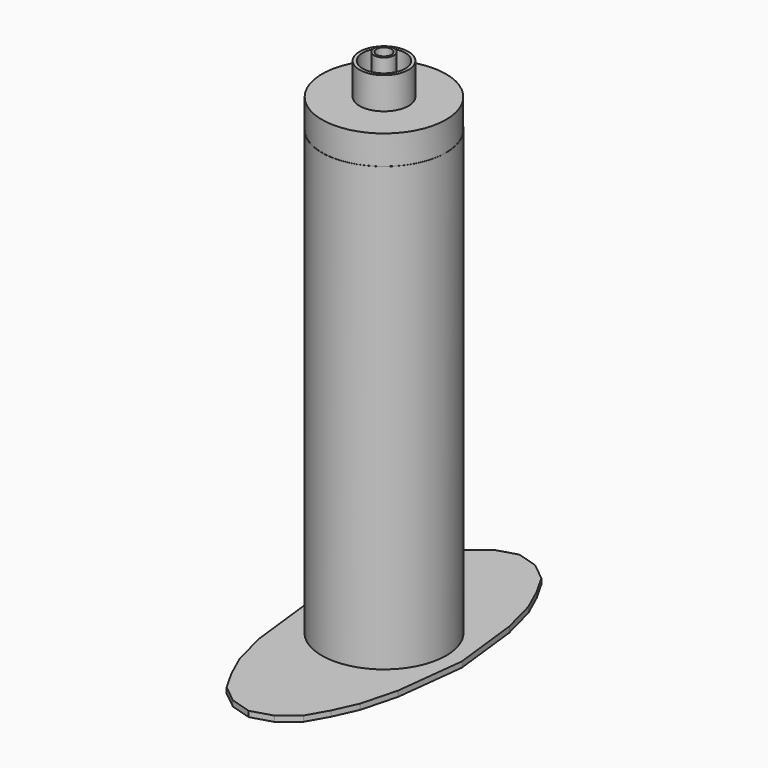
from build123d import *

# Parameters (mm, degrees)
F0_R      = 28.3177523181
F1_DEPTH  = 141.224
F2_DEPTH  = 60.452
F3_R      = 26.2473166526
F4_DEPTH  = 198.628
F5_R      = 28.3177523181
F6_DEPTH  = 2.54
F7_R      = 28.2282534547
F8_DEPTH  = 13.208
F9_R      = 11.1815753047
F10_DEPTH = 14.478
F11_R     = 9.7009276287
F12_DEPTH = 13.462
F13_R     = 4.462331727
F14_DEPTH = 14.478
F15_DEPTH = 3.556
F16_R     = 3.4559757879
F17_DEPTH = 18.034


# Not quite as in the source:
# - a feature names something its author has since deleted; it is built from what else it names


with BuildPart() as f1:
    # F0 (on Top) → F1 (new body)
    with BuildSketch(Plane.XY):
        Circle(F0_R)
    extrude(amount=F1_DEPTH)

    # F2 (add): a face of the model
    f2_faces = [f1.faces().sort_by_distance(p)[0] for p in [
        (0, 0, 0),
    ]]
    extrude(f2_faces, amount=F2_DEPTH)

    # F3 (on face) → F4 (cut)
    with BuildSketch(Plane(origin=(0, 0, -60.452), x_dir=(1, 0, 0), z_dir=(0, 0, -1))):
        Circle(F3_R)
    extrude(amount=-F4_DEPTH, mode=Mode.SUBTRACT)

    # F7 (on face) → F8 (join)
    with BuildSketch(Plane.XY.offset(141.224)):
        Circle(F7_R)
    extrude(amount=F8_DEPTH)

    # F9 (on face) → F10 (join)
    with BuildSketch(Plane.XY.offset(154.432)):
        Circle(F9_R)
    extrude(amount=F10_DEPTH)

    # F11 (on face) → F12 (cut)
    with BuildSketch(Plane.XY.offset(168.91)):
        Circle(F11_R)
    extrude(amount=-F12_DEPTH, mode=Mode.SUBTRACT)

    # F13 (on face) → F14 (join)
    with BuildSketch(Plane.XY.offset(168.91)):
        Circle(F13_R)
    extrude(amount=-F14_DEPTH)

    # F15 (add): a face of the model
    f15_faces = [f1.faces().sort_by_distance(p)[0] for p in [
        (0, 0, 168.91),
    ]]
    extrude(f15_faces, amount=F15_DEPTH)

    # F16 (on face) → F17 (cut)
    with BuildSketch(Plane.XY.offset(172.466)):
        Circle(F16_R)
    extrude(amount=-F17_DEPTH, mode=Mode.SUBTRACT)


with BuildPart() as f6:
    # F5 (on face) → F6 (new body)
    with BuildSketch(Plane(origin=(0, 0, -60.452), x_dir=(1, 0, 0), z_dir=(0, 0, -1))):
        Polygon((9.4713624567, 74.2058157921), (0, 77.0585462451), (-9.4713624567, 74.2058157921), (-17.4607206136, 67.7697062492), (-22.6705633104, 58.6060807109), (-27.5022350252, 47.904137522), (-31.7738913, 31.6246189177), (-35.4287400842, 0), (-31.7738913, -31.6246189177), (-27.5022350252, -47.904137522), (-22.6705633104, -58.6060807109), (-17.4607206136, -67.7697062492), (-9.4713624567, -74.2058157921), (0, -77.0585462451), (9.4713624567, -74.2058157921), (17.4607206136, -67.7697062492), (22.6705633104, -58.6060807109), (27.5022350252, -47.904137522), (31.7738913, -31.6246189177), (35.4287400842, 0), (31.7738913, 31.6246189177), (27.5022350252, 47.904137522), (22.6705633104, 58.6060807109), (17.4607206136, 67.7697062492), align=None)
        Circle(F5_R, mode=Mode.SUBTRACT)
    extrude(amount=F6_DEPTH)


solid = Compound([f1.part, f6.part])
